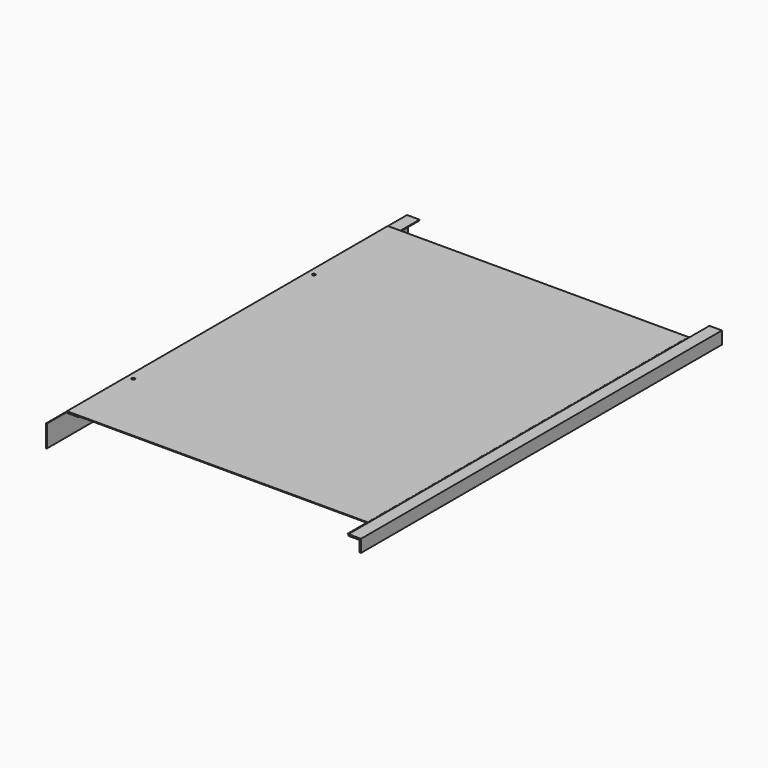
from build123d import *

# Parameters (mm, degrees)
F0_W     = 609.6
F0_H     = 863.6
F1_DEPTH = 1.5875
F3_DEPTH = 863.6
F5_DEPTH = 914.4
F4_R     = 3.175
F6_DEPTH = 25.4
F7_W     = 611.1875
F7_H     = 50.8
F8_DEPTH = 25.4


# Not quite as in the source:
# - a feature names something its author has since deleted; it is built from what else it names


with BuildPart() as f1:
    # F0 (on Top) → F1 (new body)
    with BuildSketch(Plane.XY):
        Rectangle(F0_W, F0_H)
    extrude(amount=F1_DEPTH)

    # F2 (on face) → F5 (join)
    with BuildSketch(Plane.XZ.offset(431.8)):
        Polygon((-280.9875, -1.5875), (-280.9875, 0), (-304.8, 0), (-306.3875, 0), (-306.3875, -44.45), (-304.8, -44.45), (-304.8, -1.5875), align=None)
    extrude(amount=-F5_DEPTH)

    # F4 (on face) → F6 (cut)
    with BuildSketch(Plane.XY.offset(1.5875)):
        with Locations((-292.1, 228.6)):
            Circle(F4_R)
        with Locations((-292.1, -228.6)):
            Circle(F4_R)
    extrude(amount=-F6_DEPTH, mode=Mode.SUBTRACT)

    # F7 (on face) → F8 (cut)
    with BuildSketch(Plane.XY.offset(1.5875)):
        with Locations((0.79375, -406.4)):
            Rectangle(F7_W, F7_H)
    extrude(amount=-F8_DEPTH, mode=Mode.SUBTRACT)


with BuildPart() as f3:
    # F2 (on face) → F3 (new body, through all)
    with BuildSketch(Plane.XZ.offset(431.8)):
        with BuildLine():
            ThreePointArc((304.8, 1.5875), (305.59375, 0.79375), (306.3875, 1.5875))
            ThreePointArc((306.3875, 1.5875), (305.59375, 2.38125), (304.8, 1.5875))
        make_face()
    extrude(amount=-F3_DEPTH)


with BuildPart() as f5:
    # F2 (on face) → F5, piece 2 (new body)
    with BuildSketch(Plane.XZ.offset(431.8)):
        Polygon((331.7875, 1.5875), (306.3875, 1.5875), (306.3875, -1.5875), (328.6125, -1.5875), (328.6125, -23.8125), (331.7875, -23.8125), align=None)
    extrude(amount=-F5_DEPTH)


solid = Compound([f1.part, f3.part, f5.part])
